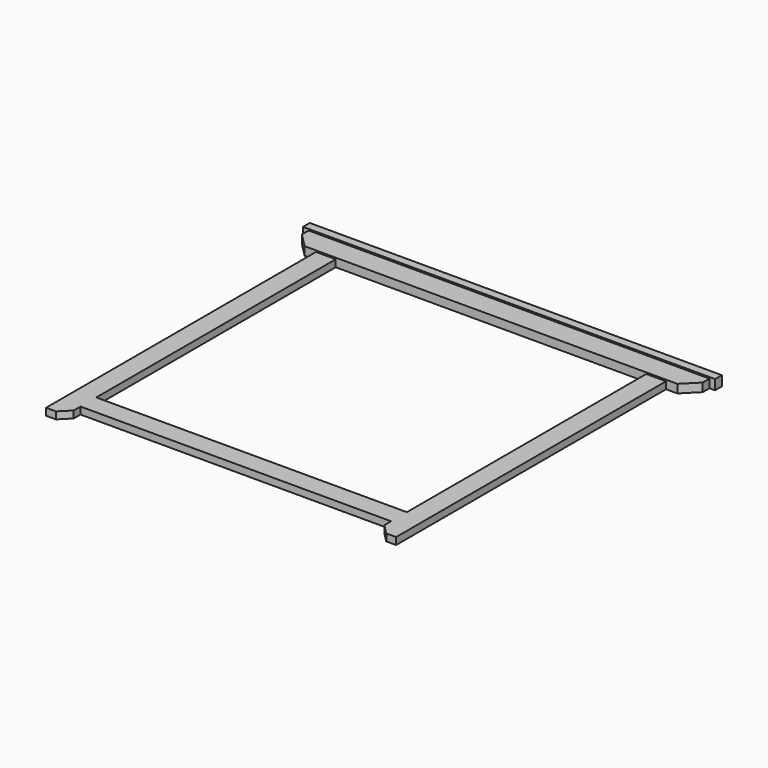
from build123d import *

# Parameters (mm, degrees)
F1_DEPTH = 30
F0_W     = 20
F0_H     = 30
F0_W_2   = 1420
F2_DEPTH = 35
F0_W_3   = 1100
F0_H_2   = 70
F3_DEPTH = 25


with BuildPart() as f1:
    # F0 (on Top) → F1 (new body)
    with BuildSketch(Plane.XY):
        Polygon((-1947.5297451019, -160.4416549206), (-1877.5297451019, -160.4416549206), (-777.5297451019, -160.4416549206), (-707.5297451019, -160.4416549206), (-667.5297451019, -160.4416549206), (-617.5297451019, -110.4416549206), (-617.5297451019, -80.4416549206), (-2037.5297451019, -80.4416549206), (-2037.5297451019, -110.4416549206), (-1987.5297451019, -160.4416549206), align=None)
    extrude(amount=F1_DEPTH)

    # F0 (on Top) → F2 (join)
    with BuildSketch(Plane.XY):
        with Locations((-2047.5297451019, -65.4416549206)):
            Rectangle(F0_W, F0_H)
        with Locations((-1327.5297451019, -65.4416549206)):
            Rectangle(F0_W_2, F0_H)
        with Locations((-607.5297451019, -65.4416549206)):
            Rectangle(F0_W, F0_H)
    extrude(amount=F2_DEPTH)

    # F0 (on Top) → F3 (join)
    with BuildSketch(Plane.XY):
        Polygon((-1877.5297451019, -1220.4416549206), (-1877.5297451019, -160.4416549206), (-1947.5297451019, -160.4416549206), (-1947.5297451019, -1355.4416549206), (-1912.5297451019, -1355.4416549206), (-1877.5297451019, -1320.4416549206), (-1877.5297451019, -1290.4416549206), align=None)
        with Locations((-1327.5297451019, -1255.4416549206)):
            Rectangle(F0_W_3, F0_H_2)
        Polygon((-707.5297451019, -160.4416549206), (-777.5297451019, -160.4416549206), (-777.5297451019, -1220.4416549206), (-777.5297451019, -1290.4416549206), (-777.5297451019, -1320.4416549206), (-742.5297451019, -1355.4416549206), (-707.5297451019, -1355.4416549206), align=None)
    extrude(amount=F3_DEPTH)


solid = f1.part
